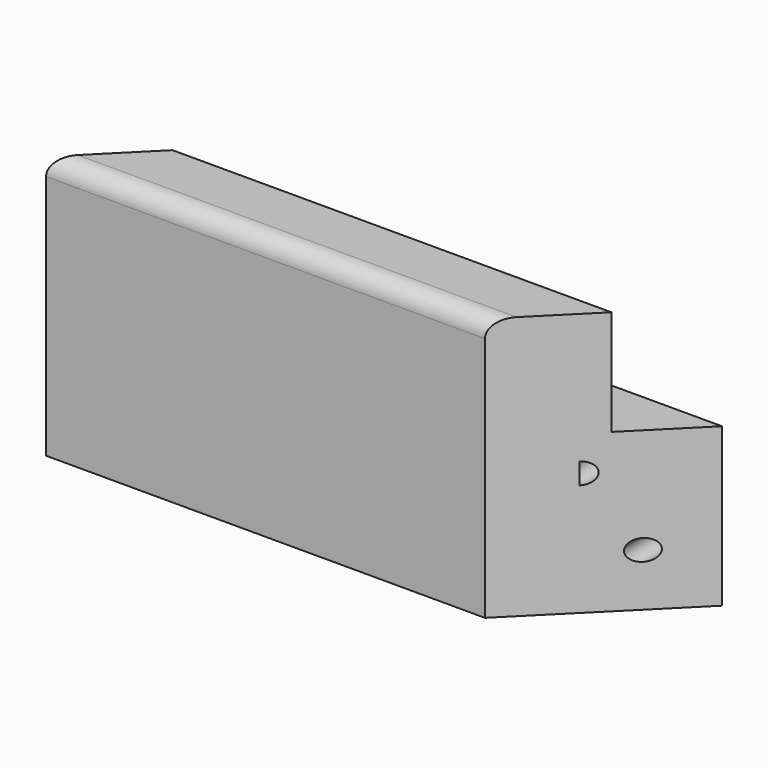
from build123d import *

# Parameters (mm, degrees)
F3_DEPTH = 165
F4_SIZE  = 79.99999
F5_R     = 6
F6_DEPTH = 50
F7_W     = 116
F7_H     = 90
F8_DEPTH = 5
F9_R     = 10


# Not quite as in the source:
# - a fillet or chamfer is up to 0.001 mm smaller than in the source, because OpenCascade refuses the exact size


with BuildPart() as f3:
    # F2 (on Right) → F3 (new body, symmetric)
    with BuildSketch(Plane.YZ):
        Polygon((-40, 75), (-40, -75), (40, -75), (40, 15), (0, 15), (0, 75), align=None)
    extrude(amount=F3_DEPTH, both=True)

    # F4 (size 80 in the source; OpenCascade refuses exactly that, so slightly less here)
    f4_edges = [f3.edges().sort_by_distance(p)[0] for p in [
        (-165, 40, -30),
        (165, -40, 0),
    ]]
    chamfer(f4_edges, length=F4_SIZE)

    # F5 (on face) → F6 (cut)
    with BuildSketch(Plane(origin=(0, 40, 0), x_dir=(-1, 0, 0), z_dir=(0, 1, 0))):
        with Locations((35, -5)):
            Circle(F5_R)
        with Locations((55, -45)):
            Circle(F5_R)
        with Locations((-115, -5)):
            Circle(F5_R)
        with Locations((-135, -45)):
            Circle(F5_R)
    extrude(amount=-F6_DEPTH, mode=Mode.SUBTRACT)

    # F7 (on face) → F8 (cut)
    with BuildSketch(Plane(origin=(0, 40, 0), x_dir=(-1, 0, 0), z_dir=(0, 1, 0))):
        with Locations((67, -30)):
            Rectangle(F7_W, F7_H)
        with Locations((-147, -30)):
            Rectangle(F7_W, F7_H)
    extrude(amount=-F8_DEPTH, mode=Mode.SUBTRACT)

    # F9
    f9_edges = [f3.edges().sort_by_distance(p)[0] for p in [
        (-39.999995, -40, 75),
    ]]
    fillet(f9_edges, radius=F9_R)


solid = f3.part
